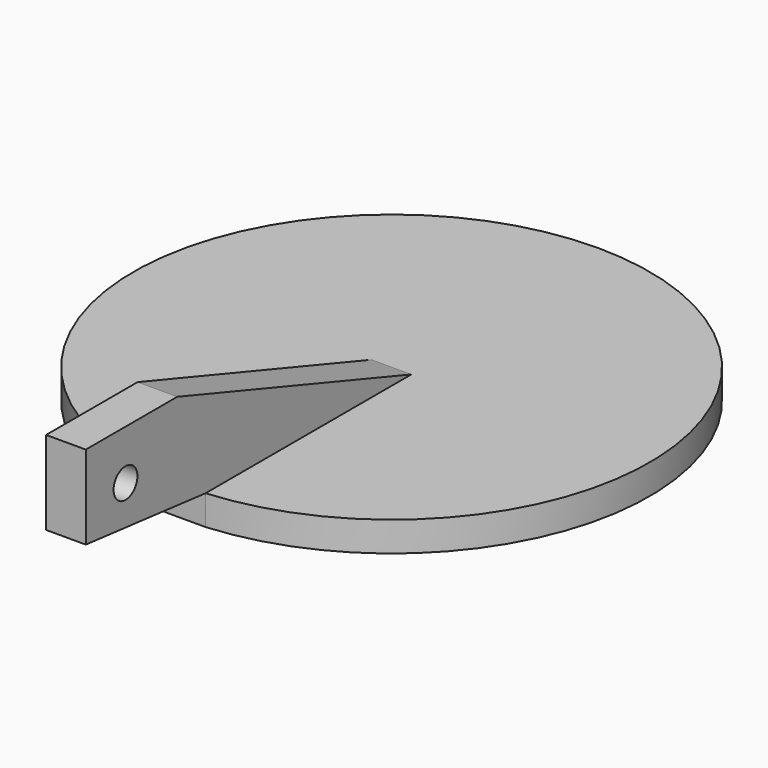
from build123d import *

# Parameters (mm, degrees)
F1_DEPTH  = 3
F3_DEPTH  = 10
F5_DEPTH  = 25
F6_W      = 4.4599839021
F6_H      = 15.0388356149
F6_W_2    = 4
F7_DEPTH  = 3
F8_R      = 1.5
F9_DEPTH  = 25
F11_DEPTH = 25


with BuildPart() as f1:
    # F0 (on Top) → F1 (new body)
    with BuildSketch(Plane.XY):
        with BuildLine():
            Line((1.9915475706, -41), (1.9915475706, -25.9236135266))
            ThreePointArc((1.9915475706, -25.9236135266), (0.0084775482, 25.9999986179), (-2.0084524294, -25.9223092883))
            Line((-2.0084524294, -25.9223092883), (-2.0084524294, -41))
            Line((-2.0084524294, -41), (1.9915475706, -41))
        make_face()
    extrude(amount=-F1_DEPTH)

    # F2 (on face) → F3 (join)
    with BuildSketch(Plane.XY):
        with BuildLine():
            Line((1.9915475706, 0), (-2.0153727382, 0))
            Line((-2.0153727382, 0), (-2.0153727382, -25.9217721756))
            ThreePointArc((-2.0153727382, -25.9217721756), (-2.0119126018, -25.9220409629), (-2.0084524294, -25.9223092883))
            Line((-2.0084524294, -25.9223092883), (-2.0084524294, -41))
            Line((-2.0084524294, -41), (1.9915475706, -41))
            Line((1.9915475706, -41), (1.9915475706, -25.9236135266))
            Line((1.9915475706, -25.9236135266), (1.9915475706, 0))
        make_face()
    extrude(amount=F3_DEPTH)

    # F4 (on face) → F5 (cut)
    with BuildSketch(Plane.YZ.offset(1.9915475706)):
        Polygon((-29.4827464968, 10), (0, 0), (0, 10), align=None)
    extrude(amount=-F5_DEPTH, mode=Mode.SUBTRACT)

    # F6 (on face) → F7 (cut)
    with BuildSketch(Plane(origin=(0, 0, -3), x_dir=(1, 0, 0), z_dir=(0, 0, -1))):
        with Locations((-0.0513555715, 33.4805821925)):
            Rectangle(F6_W, F6_H)
        with Locations((-0.0084524294, 33.4805821925)):
            Rectangle(F6_W_2, F6_H)
    extrude(amount=-F7_DEPTH, mode=Mode.SUBTRACT)

    # F8 (on face) → F9 (cut)
    with BuildSketch(Plane.YZ.offset(1.9915475706)):
        with Locations((-36, 5)):
            Circle(F8_R)
    extrude(amount=-F9_DEPTH, mode=Mode.SUBTRACT)

    # F10 (on face) → F11 (cut)
    with BuildSketch(Plane.YZ.offset(1.9915475706)):
        Polygon((-25.9236135266, -3), (-25.9236135266, 0), (-41, 1.5707125422), (-41, 0), (-25.9611643851, 0), (-25.9611643851, -3), align=None)
    extrude(amount=-F11_DEPTH, mode=Mode.SUBTRACT)


solid = f1.part
